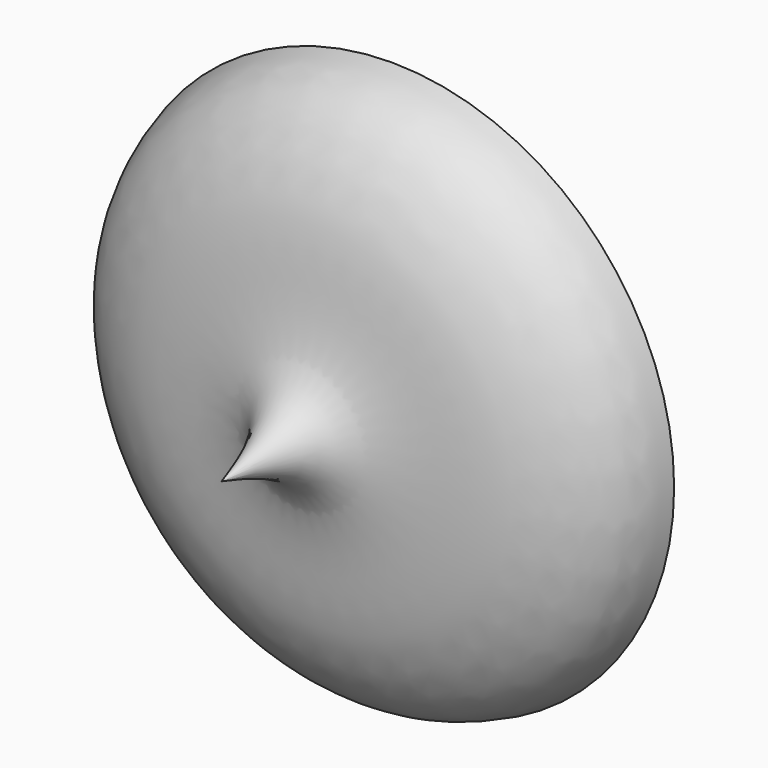
from build123d import *


# Not quite as in the source:
# - ends of sketch curves that miss each other by under 0.0002 mm in the source are joined
# - the dataset's text gives a spline's control points without its knots; the knots are read off the source's solid


with BuildPart() as f1:
    # F0 (on Top) → F1 (revolve)
    with BuildSketch(Plane.XY):
        with BuildLine():
            Line((-56.6354792879, 22.000892014), (-61.7798753083, 20.591372624))
            add(Edge.make_bspline(
                [(-61.7798753083, 20.591372624), (-60.8726611951, 17.2802662239), (-58.6643687381, 9.2205467134), (-38.5555184737, -2.7790113201), (-7.4519401131, -1.1586217978), (-2.3946793956, -18.015008946), (0, -25.9967297316)],
                knots=[0, 0, 0, 0, 0.18171084, 0.442310885, 0.7359268767, 1, 1, 1, 1], degree=3))
            Line((0, -25.9967297316), (0, -10.6937765296))
            Line((0, -10.6937765296), (0, 48.9080585539))
            Line((0, 48.9080585539), (-5.3484351374, 48.9080585539))
            add(Edge.make_bspline(
                [(-5.2015190112, 44.2038215697), (-5.222645793, 45.8382173884), (-5.2855406335, 47.3731343126), (-5.3484351374, 48.9080585539)],
                knots=[0.8943942358, 0.8943942358, 0.8943942358, 0.8943942358, 1, 1, 1, 1], degree=3))
            add(Edge.make_bspline(
                [(-5.1972059227, 42.358584707), (-5.1916361848, 42.9903534667), (-5.193762809, 43.603791495), (-5.2015190112, 44.2038215697)],
                knots=[0.8556235574, 0.8556235574, 0.8556235574, 0.8556235574, 0.8943942358, 0.8943942358, 0.8943942358, 0.8943942358], degree=3))
            add(Edge.make_bspline(
                [(-5.230873143, 40.6552925609), (-5.2128393224, 41.2392797296), (-5.202078047, 41.8059454308), (-5.1972059227, 42.358584707)],
                knots=[0.8217089339, 0.8217089339, 0.8217089339, 0.8217089339, 0.8556235574, 0.8556235574, 0.8556235574, 0.8556235574], degree=3))
            add(Edge.make_bspline(
                [(-5.2988236109, 39.0229672201), (-5.2695184927, 39.5829262627), (-5.2472112351, 40.1262179758), (-5.230873143, 40.6552925609)],
                knots=[0.7909833182, 0.7909833182, 0.7909833182, 0.7909833182, 0.8217089339, 0.8217089339, 0.8217089339, 0.8217089339], degree=3))
            add(Edge.make_bspline(
                [(-5.3962027795, 37.461616099), (-5.3790526175, 37.6991086906), (-5.343229068, 38.2276593374), (-5.3135501067, 38.7415749243), (-5.2988236109, 39.0229672201)],
                knots=[0.7631997406, 0.7631997406, 0.7631997406, 0.7631997406, 0.7755429897, 0.7909833182, 0.7909833182, 0.7909833182, 0.7909833182], degree=3))
            add(Edge.make_bspline(
                [(-5.5108853745, 36.0422022641), (-5.4678439096, 36.524482473), (-5.4296715732, 36.998145809), (-5.3962027795, 37.461616099)],
                knots=[0.7391117083, 0.7391117083, 0.7391117083, 0.7391117083, 0.7631997406, 0.7631997406, 0.7631997406, 0.7631997406], degree=3))
            add(Edge.make_bspline(
                [(-25.888593997, 3.4676403055), (-22.6147563484, 4.3712970252), (-15.491289179, 6.3339288179), (-8.0783119386, 18.2327498414), (-5.985186165, 30.7276553449), (-5.5108853745, 36.0422022641)],
                knots=[0, 0, 0, 0, 0.2176988833, 0.4736706314, 0.7391117083, 0.7391117083, 0.7391117083, 0.7391117083], degree=3))
            add(Edge.make_bspline(
                [(-56.6354792879, 22.000892014), (-56.3234402148, 20.8620268255), (-55.8916040956, 19.3032009186), (-55.2286182637, 17.5024874386), (-54.6571530898, 16.2644201264), (-54.0863837231, 15.29330558), (-53.5432739623, 14.5265675979), (-52.9332461827, 13.7628475149), (-51.9773556744, 12.7487396461), (-50.5415938571, 11.4961152709), (-48.8416949703, 10.2514755417), (-46.9050057964, 9.051510852), (-44.759176956, 7.9269502278), (-42.4316699632, 6.9046740964), (-40.3634175586, 6.1580449153), (-38.6446133729, 5.6347975003), (-37.3274952679, 5.2819433443), (-35.9822989083, 4.9710607636), (-34.577985645, 4.6914180244), (-33.1286562953, 4.4399861747), (-31.142218448, 4.135161182), (-28.7327790262, 3.818409007), (-26.7869447617, 3.580255968), (-25.888593997, 3.4676403055)],
                knots=[0, 0, 0, 0, 0.0625, 0.09375, 0.125, 0.15625, 0.171875, 0.1875, 0.21875, 0.25, 0.28125, 0.3125, 0.34375, 0.375, 0.40625, 0.421875, 0.4375, 0.453125, 0.46875, 0.484375, 0.5, 0.53125, 0.557702776, 0.557702776, 0.557702776, 0.557702776], degree=3))
        make_face()
        with BuildLine():
            Line((-18.1149467827, 36.0422022641), (-5.5108853745, 36.0422022641))
            add(Edge.make_bspline(
                [(-5.5108853745, 36.0422022641), (-5.4678439096, 36.524482473), (-5.4296715732, 36.998145809), (-5.3962027795, 37.461616099)],
                knots=[0.7391117083, 0.7391117083, 0.7391117083, 0.7391117083, 0.7631997406, 0.7631997406, 0.7631997406, 0.7631997406], degree=3))
            Line((-5.3962027795, 37.461616099), (-18.1149467827, 37.461616099))
            Line((-18.1149467827, 37.461616099), (-18.1149467827, 36.0422022641))
        make_face()
        with BuildLine():
            add(Edge.make_bspline(
                [(-5.1972059227, 42.358584707), (-5.1916361848, 42.9903534667), (-5.193762809, 43.603791495), (-5.2015190112, 44.2038215697)],
                knots=[0.8556235574, 0.8556235574, 0.8556235574, 0.8556235574, 0.8943942358, 0.8943942358, 0.8943942358, 0.8943942358], degree=3))
            Line((-5.2015190112, 44.2038215697), (-17.9730057716, 44.2038215697))
            Line((-17.9730057716, 44.2038215697), (-17.9730057716, 42.358584707))
            Line((-17.9730057716, 42.358584707), (-5.1972059227, 42.358584707))
        make_face()
        with BuildLine():
            Line((-18.0439762771, 39.0229672201), (-5.2988236109, 39.0229672201))
            add(Edge.make_bspline(
                [(-5.2988236109, 39.0229672201), (-5.2695184927, 39.5829262627), (-5.2472112351, 40.1262179758), (-5.230873143, 40.6552925609)],
                knots=[0.7909833182, 0.7909833182, 0.7909833182, 0.7909833182, 0.8217089339, 0.8217089339, 0.8217089339, 0.8217089339], degree=3))
            Line((-5.230873143, 40.6552925609), (-18.0439762771, 40.6552925609))
            Line((-18.0439762771, 40.6552925609), (-18.0439762771, 39.0229672201))
        make_face()
    revolve(axis=Axis((0, 19.1071410121, 0), (0, -1, 0)))


solid = f1.part
